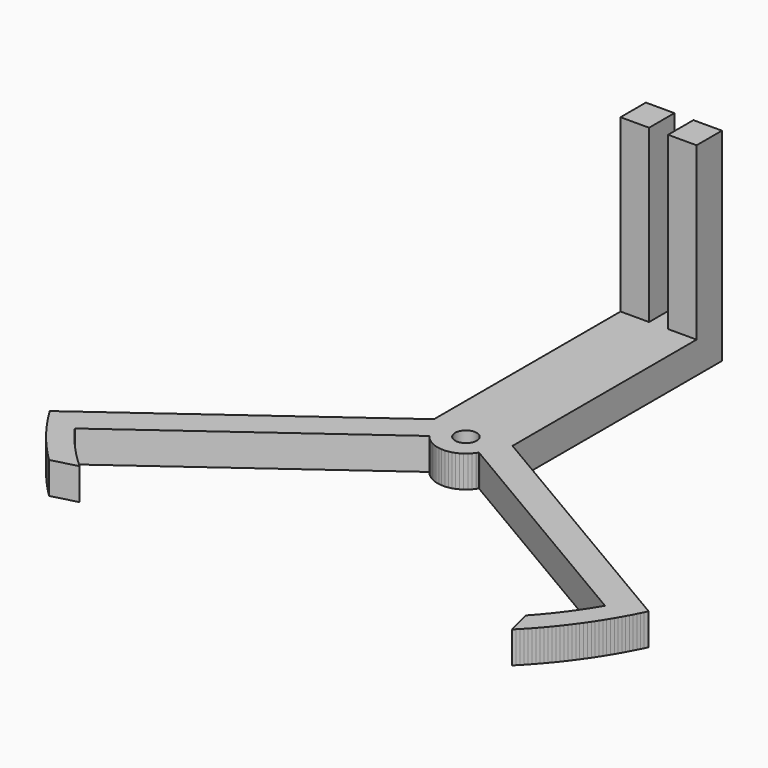
from build123d import *

# Parameters (mm, degrees)
F0_R     = 1.7
F0_W     = 3
F0_H     = 5
F1_DEPTH = 5
F0_W_2   = 4.5
F2_DEPTH = 32


# Not quite as in the source:
# - a feature names something its author has since deleted; it is built from what else it names


with BuildPart() as f1:
    # F0 (on Top) → F1 (new body)
    with BuildSketch(Plane.XY):
        with BuildLine():
            Line((-37.42359, -20.713661), (-33.444589, -19.664665))
            Line((-33.444589, -19.664665), (-33.814619, -19.328399))
            Line((-33.814619, -19.328399), (-34.181145, -18.988316))
            Line((-34.181145, -18.988316), (-34.544128, -18.644454))
            Line((-34.544128, -18.644454), (-34.903529, -18.29685))
            Line((-34.903529, -18.29685), (-35.259309, -17.94554))
            Line((-35.259309, -17.94554), (-35.611429, -17.590562))
            Line((-35.611429, -17.590562), (-35.959853, -17.231955))
            Line((-35.959853, -17.231955), (-36.304542, -16.869758))
            Line((-36.304542, -16.869758), (-36.645459, -16.504008))
            Line((-36.645459, -16.504008), (-36.982569, -16.134745))
            Line((-36.982569, -16.134745), (-37.315835, -15.76201))
            Line((-37.315835, -15.76201), (-37.64522, -15.385841))
            Line((-37.64522, -15.385841), (-37.97069, -15.00628))
            Line((-37.97069, -15.00628), (-38.29221, -14.623366))
            Line((-38.29221, -14.623366), (-38.609746, -14.237142))
            Line((-38.609746, -14.237142), (-38.923262, -13.847648))
            Line((-38.923262, -13.847648), (-39.232726, -13.454927))
            Line((-39.232726, -13.454927), (-39.538104, -13.059021))
            Line((-39.538104, -13.059021), (-39.839363, -12.659971))
            Line((-39.839363, -12.659971), (-40.136472, -12.257822))
            Line((-40.136472, -12.257822), (-40.199223, -12.171758))
            Line((-40.199223, -12.171758), (-4.815801, 13.567638))
            Line((-4.815801, 13.567638), (-4.499835, 13.180458))
            Line((-4.499835, 13.180458), (-4.142886, 12.8307))
            Line((-4.142886, 12.8307), (-3.749356, 12.522679))
            Line((-3.749356, 12.522679), (-3.324099, 12.260193))
            Line((-3.324099, 12.260193), (-2.872359, 12.046479))
            Line((-2.872359, 12.046479), (-2.399707, 11.884173))
            Line((-2.399707, 11.884173), (-1.911973, 11.775276))
            Line((-1.911973, 11.775276), (-1.415172, 11.721133))
            Line((-1.415172, 11.721133), (-0.91543, 11.72241))
            Line((-0.91543, 11.72241), (-0.418912, 11.779092))
            Line((-0.418912, 11.779092), (0.068259, 11.890479))
            Line((0.068259, 11.890479), (0.540075, 12.055198))
            Line((0.540075, 12.055198), (0.990717, 12.271218))
            Line((0.990717, 12.271218), (1.414627, 12.535874))
            Line((1.414627, 12.535874), (1.806578, 12.845903))
            Line((1.806578, 12.845903), (2.161735, 13.19748))
            Line((2.161735, 13.19748), (2.475718, 13.58627))
            Line((2.475718, 13.58627), (2.5697381369, 13.7302913689))
            Line((2.5697381369, 13.7302913689), (1.9580461126, 13.7302913689))
            ThreePointArc((1.9580461126, 13.7302913689), (-1.176782, 12.214814), (-4.3116101126, 13.7302913689))
            Line((-4.3116101126, 13.7302913689), (-7.176782, 13.7302913689))
            Line((-7.176782, 13.7302913689), (-7.176782, 17.4148470867))
            Line((-7.176782, 17.4148470867), (-45.510085, -10.470418))
            Line((-45.510085, -10.470418), (-45.250166, -10.897548))
            Line((-45.250166, -10.897548), (-44.986132, -11.322146))
            Line((-44.986132, -11.322146), (-44.718008, -11.744174))
            Line((-44.718008, -11.744174), (-44.445818, -12.163591))
            Line((-44.445818, -12.163591), (-44.169588, -12.580359))
            Line((-44.169588, -12.580359), (-43.889344, -12.994438))
            Line((-43.889344, -12.994438), (-43.605112, -13.405789))
            Line((-43.605112, -13.405789), (-43.316919, -13.814376))
            Line((-43.316919, -13.814376), (-43.024791, -14.220158))
            Line((-43.024791, -14.220158), (-42.728755, -14.623099))
            Line((-42.728755, -14.623099), (-42.428841, -15.02316))
            Line((-42.428841, -15.02316), (-42.125074, -15.420305))
            Line((-42.125074, -15.420305), (-41.817484, -15.814496))
            Line((-41.817484, -15.814496), (-41.5061, -16.205696))
            Line((-41.5061, -16.205696), (-41.19095, -16.59387))
            Line((-41.19095, -16.59387), (-40.872064, -16.97898))
            Line((-40.872064, -16.97898), (-40.549472, -17.360991))
            Line((-40.549472, -17.360991), (-40.223203, -17.739867))
            Line((-40.223203, -17.739867), (-39.893289, -18.115572))
            Line((-39.893289, -18.115572), (-39.55976, -18.488072))
            Line((-39.55976, -18.488072), (-39.222648, -18.857333))
            Line((-39.222648, -18.857333), (-38.881982, -19.223318))
            Line((-38.881982, -19.223318), (-38.537797, -19.585995))
            Line((-38.537797, -19.585995), (-38.190123, -19.945329))
            Line((-38.190123, -19.945329), (-37.838993, -20.301287))
            Line((-37.838993, -20.301287), (-37.484441, -20.653835))
            Line((-37.484441, -20.653835), (-37.42359, -20.713661))
        make_face()
        with BuildLine():
            Line((-3.823958, 19.853833), (-7.176782, 17.4148470867))
            Line((-7.176782, 17.4148470867), (-7.176782, 13.7302913689))
            Line((-7.176782, 13.7302913689), (-4.3116101126, 13.7302913689))
            ThreePointArc((-4.3116101126, 13.7302913689), (-2.4922073209, 19.9923338511), (2.823218, 16.214814))
            ThreePointArc((2.823218, 16.214814), (2.6007378511, 14.8993886791), (1.9580461126, 13.7302913689))
            Line((1.9580461126, 13.7302913689), (2.5697381369, 13.7302913689))
            Line((2.5697381369, 13.7302913689), (2.699204, 13.928609))
            Line((2.699204, 13.928609), (3.0354278194, 13.7302913689))
            Line((3.0354278194, 13.7302913689), (4.823218, 13.7302913689))
            Line((4.823218, 13.7302913689), (4.823218, 17.9002620213))
            Line((4.823218, 17.9002620213), (1.109423, 20.0908))
            Line((1.109423, 20.0908), (0.665545, 20.320399))
            Line((0.665545, 20.320399), (0.198946, 20.499364))
            Line((0.198946, 20.499364), (-0.284619, 20.625488))
            Line((-0.284619, 20.625488), (-0.779188, 20.697215))
            Line((-0.779188, 20.697215), (-1.27866, 20.713661))
            Line((-1.27866, 20.713661), (-1.776876, 20.674622))
            Line((-1.776876, 20.674622), (-2.267691, 20.580581))
            Line((-2.267691, 20.580581), (-2.745051, 20.432696))
            Line((-2.745051, 20.432696), (-3.20307, 20.232793))
            Line((-3.20307, 20.232793), (-3.636099, 19.983336))
            Line((-3.636099, 19.983336), (-3.823958, 19.853833))
        make_face()
        Polygon((4.823218, 13.7302913689), (3.0354278194, 13.7302913689), (40.38674, -8.300937), (40.13049, -8.730279), (39.869806, -9.156942), (39.604715, -9.580881), (39.335246, -10.002051), (39.061427, -10.420406), (38.783288, -10.835901), (38.500859, -11.248493), (38.21417, -11.658135), (37.923252, -12.064786), (37.628136, -12.4684), (37.328853, -12.868934), (37.025437, -13.266346), (36.71792, -13.660593), (36.406334, -14.051633), (36.090712, -14.439423), (35.77109, -14.823922), (35.447501, -15.205088), (35.11998, -15.582882), (34.788562, -15.957261), (34.453283, -16.328186), (34.381366, -16.406751), (35.390903, -20.395946), (35.742952, -20.040897), (36.091554, -19.682463), (36.436676, -19.320678), (36.778286, -18.955574), (37.116352, -18.587187), (37.450843, -18.21555), (37.781727, -17.840698), (38.108974, -17.462667), (38.432553, -17.081492), (38.752433, -16.697207), (39.068585, -16.30985), (39.38098, -15.919456), (39.689588, -15.526061), (39.99438, -15.129703), (40.295328, -14.730418), (40.592404, -14.328244), (40.885581, -13.923219), (41.174829, -13.515379), (41.460124, -13.104763), (41.741437, -12.69141), (42.018744, -12.275358), (42.292017, -11.856646), (42.561231, -11.435313), (42.826362, -11.011398), (43.087385, -10.584942), (43.344274, -10.155983), (43.597007, -9.724561), (43.845559, -9.290718), (44.089907, -8.854494), (44.330029, -8.415928), (44.565902, -7.975063), (44.797505, -7.53194), (45.024814, -7.086599), (45.24781, -6.639083), (45.466471, -6.189433), (45.510086, -6.098405), (4.823218, 17.9002620213), align=None)
        Polygon((-7.176782, 54.214814), (-7.176782, 17.4148470867), (-3.823958, 19.853833), (-3.636099, 19.983336), (-3.20307, 20.232793), (-2.745051, 20.432696), (-2.267691, 20.580581), (-1.776876, 20.674622), (-1.27866, 20.713661), (-0.779188, 20.697215), (-0.284619, 20.625488), (0.198946, 20.499364), (0.665545, 20.320399), (1.109423, 20.0908), (4.823218, 17.9002620213), (4.823218, 54.214814), (0.323218, 54.214814), (-2.676782, 54.214814), align=None)
        with BuildLine():
            ThreePointArc((2.823218, 16.214814), (-2.4922073209, 19.9923338511), (-4.3116101126, 13.7302913689))
            Line((-4.3116101126, 13.7302913689), (1.9580461126, 13.7302913689))
            ThreePointArc((1.9580461126, 13.7302913689), (2.6007378511, 14.8993886791), (2.823218, 16.214814))
        make_face()
        with Locations((-1.176782, 16.214814)):
            Circle(F0_R, mode=Mode.SUBTRACT)
        with BuildLine():
            Line((1.9580461126, 13.7302913689), (-4.3116101126, 13.7302913689))
            ThreePointArc((-4.3116101126, 13.7302913689), (-1.176782, 12.214814), (1.9580461126, 13.7302913689))
        make_face()
        with Locations((-1.176782, 56.714814)):
            Rectangle(F0_W, F0_H)
    extrude(amount=F1_DEPTH)

    # F0 (on Top) → F2 (join)
    with BuildSketch(Plane.XY):
        with Locations((-4.926782, 56.714814)):
            Rectangle(F0_W_2, F0_H)
        with Locations((2.573218, 56.714814)):
            Rectangle(F0_W_2, F0_H)
    extrude(amount=F2_DEPTH)


solid = f1.part
